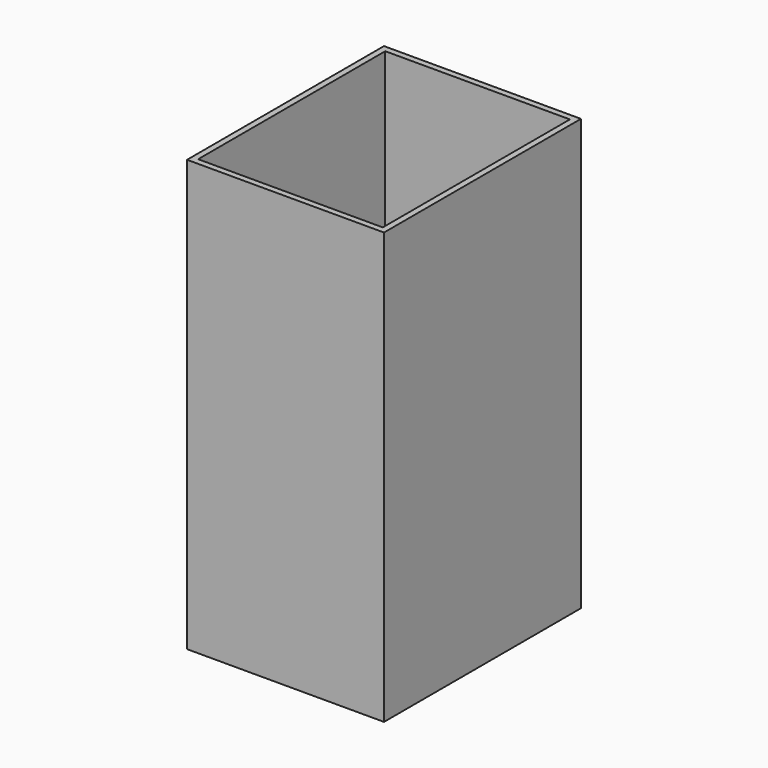
from build123d import *

# Parameters (mm, degrees)
F0_W     = 50.8
F0_H     = 63.5
F1_DEPTH = 3.175
F2_W     = 50.8
F2_H     = 63.5
F2_W_2   = 47.625
F2_H_2   = 60.325
F3_DEPTH = 107.95


# Not quite as in the source:
# - a length typed as a fraction of an inch, garbled in the dataset ("3 / 203.2 mm" for 3/8 in), is restored


with BuildPart() as f1:
    # F0 (on Top) → F1 (new body)
    with BuildSketch(Plane.XY):
        Rectangle(F0_W, F0_H)
    extrude(amount=F1_DEPTH)

    # F2 (on face) → F3 (join)
    with BuildSketch(Plane.XY.offset(3.175)):
        Rectangle(F2_W, F2_H)
        Rectangle(F2_W_2, F2_H_2, mode=Mode.SUBTRACT)
    extrude(amount=F3_DEPTH)


solid = f1.part
